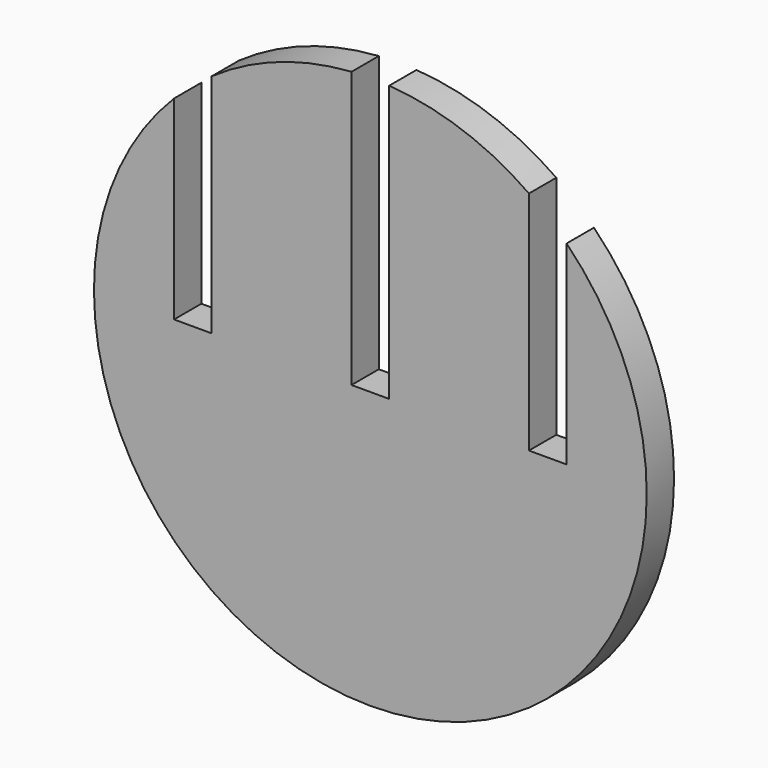
from build123d import *

# Parameters (mm, degrees)
F1_DEPTH = 3.175


# Not quite as in the source:
# - a length typed as a fraction of an inch, garbled in the dataset ("3 / 203.2 mm" for 3/8 in), is restored


with BuildPart() as f1:
    # F0 (on Front) → F1 (new body)
    with BuildSketch(Plane.XZ):
        with BuildLine():
            Line((18.25, 0), (25.7, 0))
            ThreePointArc((25.7, 0), (23.7646270747, 9.7842986463), (18.25, 18.0949578612))
            Line((18.25, 18.0949578612), (18.25, 0))
        make_face()
        with BuildLine():
            ThreePointArc((-18.25, 18.0949578612), (-23.7646270747, 9.7842986463), (-25.7, 0))
            Line((-25.7, 0), (-18.25, 0))
            Line((-18.25, 0), (-18.25, 18.0949578612))
        make_face()
        with BuildLine():
            Line((14.75, 0), (14.75, 21.0458428199))
            ThreePointArc((14.75, 21.0458428199), (8.5638701474, 24.231180906), (1.75, 25.6403490616))
            Line((1.75, 25.6403490616), (1.75, 12.8201745308))
            Line((1.75, 12.8201745308), (1.75, 0))
            Line((1.75, 0), (14.75, 0))
        make_face()
        with BuildLine():
            Line((-14.75, 0), (-1.75, 0))
            Line((-1.75, 0), (-1.75, 12.8201745308))
            Line((-1.75, 12.8201745308), (-1.75, 25.6403490616))
            ThreePointArc((-1.75, 25.6403490616), (-8.5638701474, 24.231180906), (-14.75, 21.0458428199))
            Line((-14.75, 21.0458428199), (-14.75, 0))
        make_face()
        with BuildLine():
            ThreePointArc((-25.7, 0), (-18.1726442765, -18.1726442765), (0, -25.7))
            Line((0, -25.7), (0, 0))
            Line((0, 0), (-1.75, 0))
            Line((-1.75, 0), (-14.75, 0))
            Line((-14.75, 0), (-18.25, 0))
            Line((-18.25, 0), (-25.7, 0))
        make_face()
        with BuildLine():
            ThreePointArc((0, -25.7), (18.1726442765, -18.1726442765), (25.7, 0))
            Line((25.7, 0), (18.25, 0))
            Line((18.25, 0), (14.75, 0))
            Line((14.75, 0), (1.75, 0))
            Line((1.75, 0), (0, 0))
            Line((0, 0), (0, -25.7))
        make_face()
    extrude(amount=F1_DEPTH)


solid = f1.part
